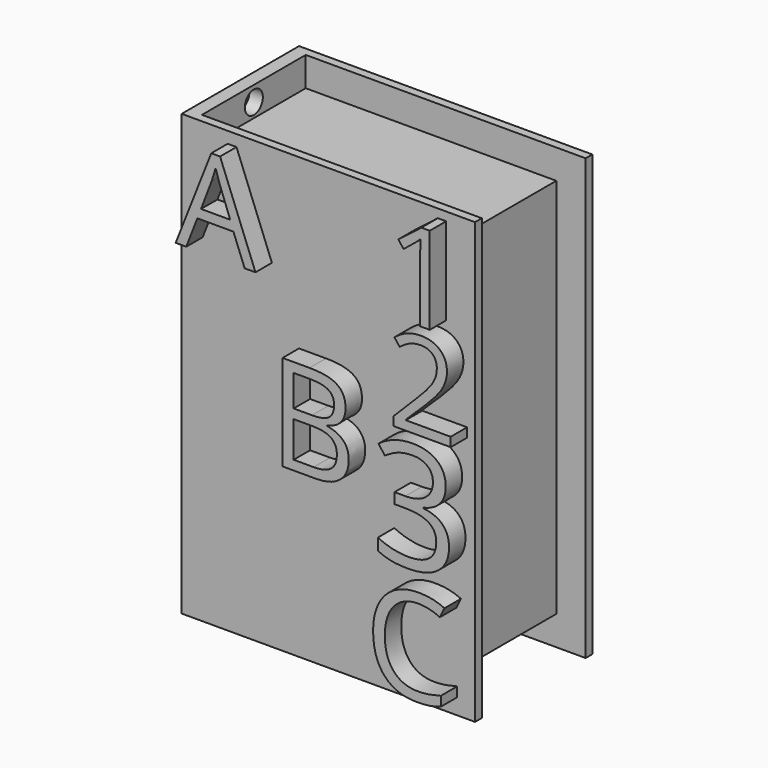
from build123d import *

# Parameters (mm, degrees)
F0_W            = 25.4
F0_H            = 38.1
F1_DEPTH        = 12.7
F2_W            = 11.2366058745
F2_H            = 38.1
F3_DEPTH        = 2.54
F4_W            = 21.6980294949
F4_H            = 11.2366058745
F5_DEPTH        = 2.54
F6_W            = 21.6916
F6_H            = 11.2366058745
F7_DEPTH        = 2.54
F10_R           = 0.9753357335
F11_DEPTH       = 25.4
F12_TEXT_SIZE   = 10.9222844345
F12_TEXT_SIZE_2 = 11.5866001426
F12_TEXT_SIZE_3 = 11.4425152511
F12_TEXT_SIZE_4 = 10.5833333333
F12_TEXT_SIZE_5 = 13.1841038118
F13_DEPTH       = 1.778


# Not quite as in the source:
# - the program builds the solid bodies; features that only make, move or delete a surface that nothing else refers to are left out
# - Text() gives the source's letters only with a copy of the font that has no kerning and outlines rounded to 1/6400 em; it was checked with that copy


with BuildPart() as f1:
    # F0 (on Front) → F1 (new body)
    with BuildSketch(Plane.XZ):
        with Locations((-12.7, 13.3949056604)):
            Rectangle(F0_W, F0_H)
    extrude(amount=F1_DEPTH)

    # F2 (on face) → F3 (cut)
    with BuildSketch(Plane.YZ):
        with Locations((-6.3450970628, 13.3949056604)):
            Rectangle(F2_W, F2_H)
    extrude(amount=-F3_DEPTH, mode=Mode.SUBTRACT)

    # F4 (on face) → F5 (cut)
    with BuildSketch(Plane.XY.offset(32.4449056604)):
        with Locations((-13.3890147474, -6.3450970628)):
            Rectangle(F4_W, F4_H)
    extrude(amount=-F5_DEPTH, mode=Mode.SUBTRACT)

    # F6 (on face) → F7 (cut)
    with BuildSketch(Plane(origin=(0, 0, -5.6550943396), x_dir=(1, 0, 0), z_dir=(0, 0, -1))):
        with Locations((-13.3858, 6.3450970628)):
            Rectangle(F6_W, F6_H)
    extrude(amount=-F7_DEPTH, mode=Mode.SUBTRACT)

    # F10 (on face) → F11 (cut)
    with BuildSketch(Plane.YZ.offset(-24.2380294949)):
        with Locations((-6.3450970628, 31.1206784099)):
            Circle(F10_R)
    extrude(amount=-F11_DEPTH, mode=Mode.SUBTRACT)

    # F12 (on face) → F13 (join)
    with BuildSketch(Plane.XZ.offset(12.7)):
        with Locations((-24.5001137571, 23.6252720502)):
            Text('A', F12_TEXT_SIZE, font='Open Sans', text_align=(TextAlign.LEFT, TextAlign.BOTTOM))
        with Locations((-16.3805053589, 9.5889882949)):
            Text('B', F12_TEXT_SIZE_2, font='Open Sans', text_align=(TextAlign.LEFT, TextAlign.BOTTOM))
        with Locations((-8.1001336005, -4.4824812645)):
            Text('C', F12_TEXT_SIZE_3, font='Open Sans', text_align=(TextAlign.LEFT, TextAlign.BOTTOM))
        with Locations((-6.191770808, 24.1448618472)):
            Text('1', F12_TEXT_SIZE_4, font='Open Sans', text_align=(TextAlign.LEFT, TextAlign.BOTTOM))
        with Locations((-6.1697526042, 15.7886581828)):
            Text('2', F12_TEXT_SIZE_4, font='Open Sans', text_align=(TextAlign.LEFT, TextAlign.BOTTOM))
        with Locations((-7.5918600884, 5.4589116956)):
            Text('3', F12_TEXT_SIZE_5, font='Open Sans', text_align=(TextAlign.LEFT, TextAlign.BOTTOM))
    extrude(amount=F13_DEPTH)


solid = f1.part
